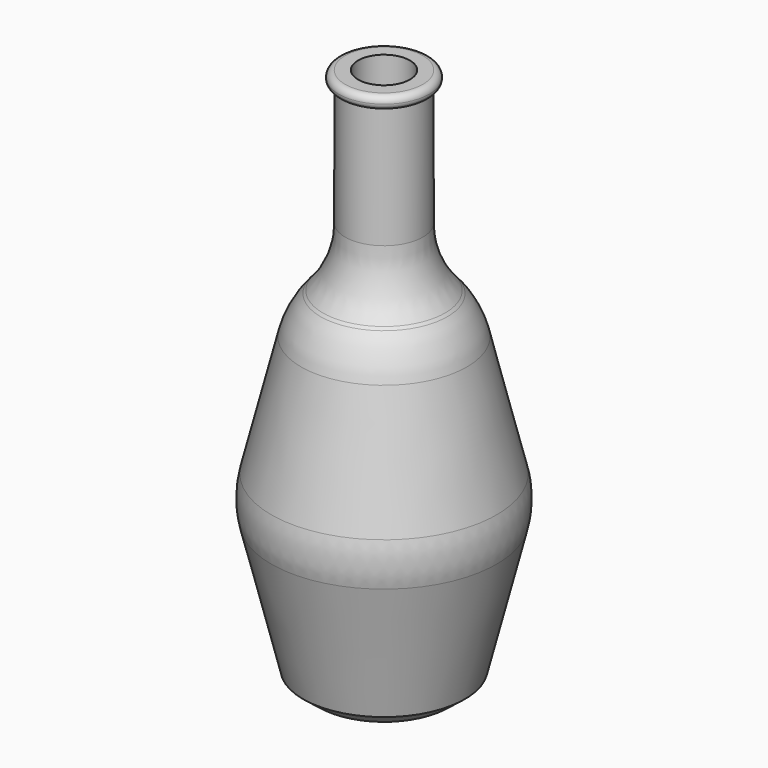
from build123d import *

# Parameters (mm, degrees)
F2_R        = 1
F3_DEPTH    = 10
F4_R        = 3.5
F4_R_2      = 2
F5_DEPTH    = 1
F6_DEPTH    = 35
F7_S5_R     = 2
F7_T6_DEPTH = 6
F8_R        = 0.49999
F9_R        = 7
F10_SIZE    = 1
F11_R       = 1
F12_DEPTH   = 35


# Not quite as in the source:
# - a fillet or chamfer that OpenCascade refuses, or shapes differently, is made with other operations: its cross-section is extruded or revolved along the edge and cut away or added
# - a fillet or chamfer is up to 0.001 mm smaller than in the source, because OpenCascade refuses the exact size


with BuildPart() as f1:
    # F0 (on Front) → F1 (revolve)
    with BuildSketch(Plane.XZ):
        Polygon((-6, 0), (0, 0), (0, 40.6942627281), (-3, 40.6942627281), (-3, 28.6942627281), (-6, 25.2438845978), (-9.1123259154, 12.6219422989), align=None)
    revolve(axis=Axis((0, 0, 20.347131364), (0, 0, -1)))

    # F2 (on Top) → F3 (cut)
    with BuildSketch(Plane.XY):
        Circle(F2_R)
    extrude(amount=F3_DEPTH, mode=Mode.SUBTRACT)

    # F4 (on face) → F5 (join)
    with BuildSketch(Plane.XY.offset(40.6942627281)):
        Circle(F4_R)
        Circle(F4_R_2, mode=Mode.SUBTRACT)
    extrude(amount=F5_DEPTH)

    # F6 (cut): a face of the model
    f6_faces = [f1.faces().sort_by_distance(p)[0] for p in [
        (0, 0, 40.6942627281),
    ]]
    extrude(f6_faces, amount=-F6_DEPTH, mode=Mode.SUBTRACT)

    # F7: chamfer of 2 on 1 edges, made by hand


with BuildPart() as f7_tool2:
    # F7_s3 → F7_t4 (revolve)
    with BuildSketch(Plane.XZ):
        Polygon((1, 3.6942627281), (3, 5.6942627281), (1, 5.6942627281), align=None)
    revolve(axis=Axis((0, 0, 5.6942627281), (0, 0, -1)))

    # F7_s5 → F7_t6 (intersect, symmetric)
    with BuildSketch(Plane.XY.offset(4.7)):
        Circle(F7_S5_R)
    extrude(amount=F7_T6_DEPTH, both=True, mode=Mode.INTERSECT)


with BuildPart() as f1_1:
    add(f1.part)

    # F7_t1: cut F7_tool2
    add(f7_tool2.part, mode=Mode.SUBTRACT)

    # F8 (radius 0.5 in the source; OpenCascade refuses exactly that, so slightly less here)
    f8_edges = [f1_1.edges().sort_by_distance(p)[0] for p in [
        (-3.5, 0, 41.694263),
        (-3.5, 0, 40.694263),
    ]]
    fillet(f8_edges, radius=F8_R)

    # F9
    f9_edges = [f1_1.edges().sort_by_distance(p)[0] for p in [
        (3, 0, 28.694263),
        (6, 0, 25.243885),
        (9.112326, 0, 12.621942),
    ]]
    fillet(f9_edges, radius=F9_R)

    # F10
    f10_edges = [f1_1.edges().sort_by_distance(p)[0] for p in [
        (6, 0, 0),
    ]]
    chamfer(f10_edges, length=F10_SIZE)

    # F11 (on face) → F12 (cut)
    with BuildSketch(Plane.XY.offset(41.6942627281)):
        with Locations((-6.5546142869, 0)):
            Circle(F11_R)
    extrude(amount=-F12_DEPTH, mode=Mode.SUBTRACT)


solid = f1_1.part
